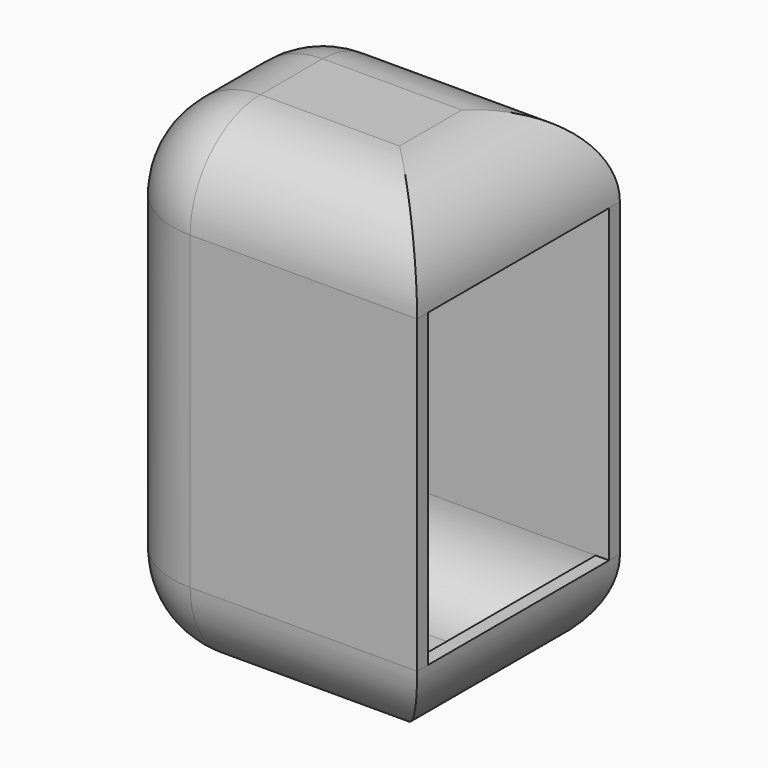
from build123d import *

# Parameters (mm, degrees)
F0_W     = 59.3015290797
F0_H     = 91.5408506989
F1_DEPTH = 47.752
F2_R     = 16.5566766108
F3_T     = -2.54


# Not quite as in the source:
# - a shell that OpenCascade refuses in one call is made with other operations: the cavity is built on its own and cut out


with BuildPart() as f1:
    # F0 (on Front) → F1 (new body)
    with BuildSketch(Plane.XZ):
        with Locations((-0.7059704512, -7.1773678064)):
            Rectangle(F0_W, F0_H)
    extrude(amount=F1_DEPTH)

    # F2
    f2_edges = [f1.edges().sort_by_distance(p)[0] for p in [
        (-30.356735, -23.876, 38.593058),
        (-30.356735, -23.876, -52.947793),
        (-30.356735, 0, -7.177368),
        (-30.356735, -47.752, -7.177368),
        (28.944794, -23.876, -52.947793),
        (-0.70597, 0, -52.947793),
        (-0.70597, -47.752, -52.947793),
        (28.944794, -23.876, 38.593058),
        (-0.70597, 0, 38.593058),
        (-0.70597, -47.752, 38.593058),
    ]]
    fillet(f2_edges, radius=F2_R)

    # F3: a shell. OpenCascade refuses it in one call, so the cavity is built on its own and cut out:
    # the body offset inwards by the wall thickness, plus a prism from it out through each open face.
    f3_core = offset(f1.part, amount=F3_T, mode=Mode.PRIVATE)
    f3_exits = [f3_core.faces().sort_by_distance(p)[0] for p in [
        (26.404794, -23.876, -7.177368),
    ]]
    add(f3_core, mode=Mode.SUBTRACT)
    extrude(f3_exits, amount=-F3_T, mode=Mode.SUBTRACT)


solid = f1.part
